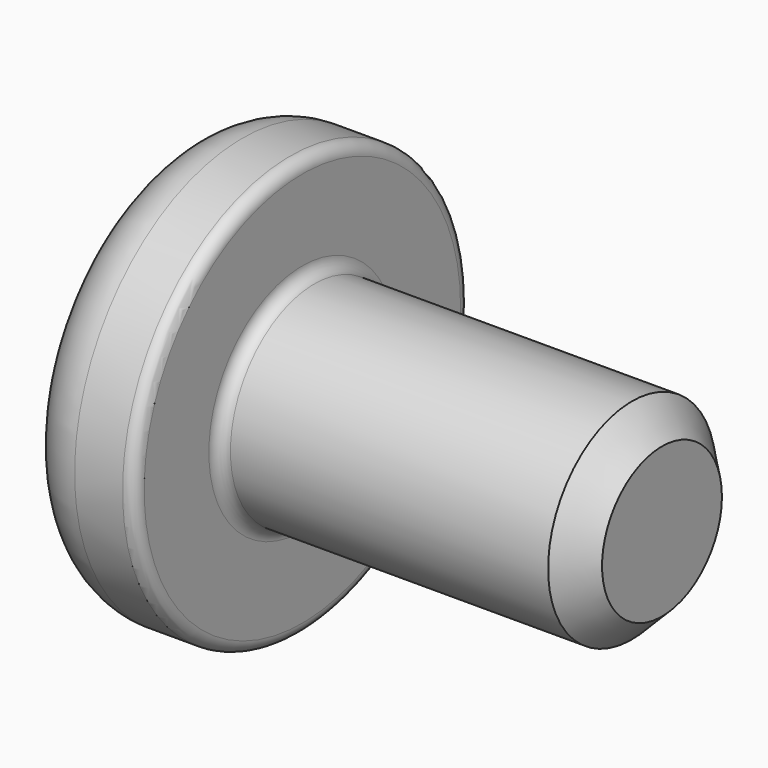
from build123d import *

# Parameters (mm, degrees)
F2_SIZE  = 0.5
F3_R     = 0.2
F4_R     = 0.2
F5_R     = 1
F7_DEPTH = 1.5
F8_SIZE  = 1.49999


# Not quite as in the source:
# - a fillet or chamfer is up to 0.001 mm smaller than in the source, because OpenCascade refuses the exact size


with BuildPart() as f1:
    # F0 (on Top) → F1 (revolve)
    with BuildSketch(Plane.XY):
        Polygon((0, 3.5), (0, 0), (8, 0), (8, 1.75), (2, 1.75), (2, 3.5), align=None)
    revolve(axis=Axis((4, 0, 0), (-1, 0, 0)))

    # F2
    f2_edges = [f1.edges().sort_by_distance(p)[0] for p in [
        (8, -1.75, 0),
    ]]
    chamfer(f2_edges, length=F2_SIZE)

    # F3
    f3_edges = [f1.edges().sort_by_distance(p)[0] for p in [
        (2, -1.75, 0),
    ]]
    fillet(f3_edges, radius=F3_R)

    # F4
    f4_edges = [f1.edges().sort_by_distance(p)[0] for p in [
        (2, -3.5, 0),
    ]]
    fillet(f4_edges, radius=F4_R)

    # F5
    f5_edges = [f1.edges().sort_by_distance(p)[0] for p in [
        (0, -3.5, 0),
    ]]
    fillet(f5_edges, radius=F5_R)

    # F6 (on face) → F7 (cut)
    with BuildSketch(Plane(origin=(0, 0, 0), x_dir=(0, -1, 0), z_dir=(-1, 0, 0))):
        Polygon((-0.75, 2.25), (-0.75, 0.75), (-2.25, 0.75), (-2.25, -0.75), (-0.75, -0.75), (-0.75, -2.25), (0.75, -2.25), (0.75, -0.75), (2.25, -0.75), (2.25, 0.75), (0.75, 0.75), (0.75, 2.25), align=None)
    extrude(amount=-F7_DEPTH, mode=Mode.SUBTRACT)

    # F8 (size 1.5 in the source; OpenCascade refuses exactly that, so slightly less here)
    f8_edges = [f1.edges().sort_by_distance(p)[0] for p in [
        (1.5, 2.25, 0),
        (1.5, 0, 2.25),
        (1.5, 0, -2.25),
        (1.5, -2.25, 0),
    ]]
    chamfer(f8_edges, length=F8_SIZE)


solid = f1.part
